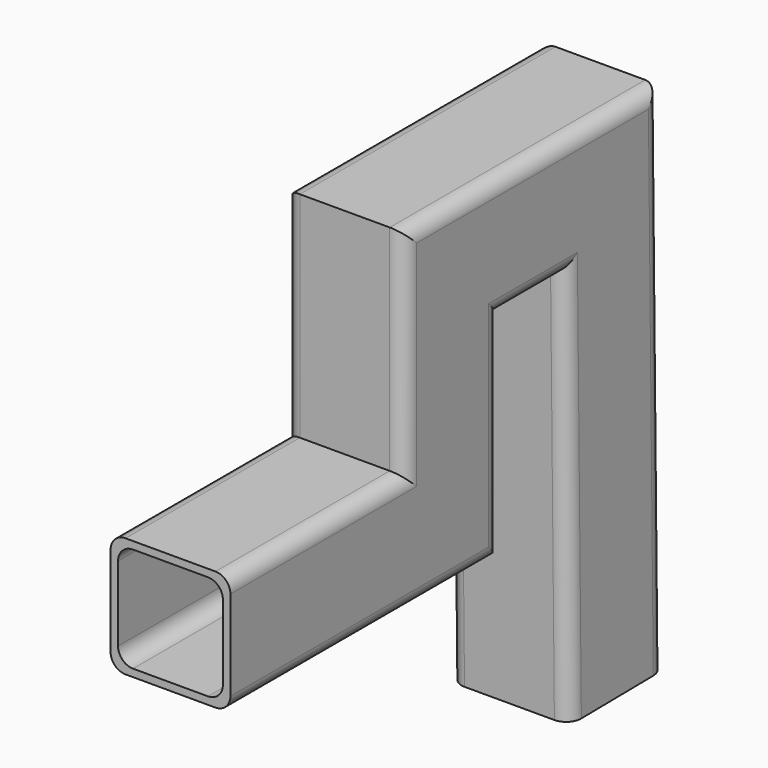
from build123d import *


with BuildPart() as f2:
    # F2: sweep along a path in F1
    with BuildLine(Plane.YZ) as f2_path:
        Line((0, 0), (235.4986518621, 0))
        Line((235.4986518621, 0), (235.4986518621, 181.7011833191))
        Line((235.4986518621, 181.7011833191), (405.3635597229, 181.7011833191))
        Line((405.3635597229, 181.7011833191), (410.0448787212, -205.5106014013))
    # F0 (on Front) → F2 (sweep)
    with BuildSketch(Plane.XZ):
        with BuildLine():
            Line((-43.4998961684, 38.1), (-43.4998961684, -38.1))
            ThreePointArc((-43.4998961684, -38.1), (-39.7801522895, -47.0802561211), (-30.7998961684, -50.8))
            Line((-30.7998961684, -50.8), (45.4001038316, -50.8))
            ThreePointArc((45.4001038316, -50.8), (54.3803599527, -47.0802561211), (58.1001038316, -38.1))
            Line((58.1001038316, -38.1), (58.1001038316, 38.1))
            ThreePointArc((58.1001038316, 38.1), (54.3803599527, 47.0802561211), (45.4001038316, 50.8))
            Line((45.4001038316, 50.8), (-30.7998961684, 50.8))
            ThreePointArc((-30.7998961684, 50.8), (-39.7801522895, 47.0802561211), (-43.4998961684, 38.1))
        make_face()
        with BuildLine():
            ThreePointArc((-37.1498961684, 31.75), (-33.4301522895, 40.7302561211), (-24.4498961684, 44.45))
            Line((-24.4498961684, 44.45), (39.0501038316, 44.45))
            ThreePointArc((39.0501038316, 44.45), (48.0303599527, 40.7302561211), (51.7501038316, 31.75))
            Line((51.7501038316, 31.75), (51.7501038316, -31.75))
            ThreePointArc((51.7501038316, -31.75), (48.0303599527, -40.7302561211), (39.0501038316, -44.45))
            Line((39.0501038316, -44.45), (-24.4498961684, -44.45))
            ThreePointArc((-24.4498961684, -44.45), (-33.4301522895, -40.7302561211), (-37.1498961684, -31.75))
            Line((-37.1498961684, -31.75), (-37.1498961684, 31.75))
        make_face(mode=Mode.SUBTRACT)
    sweep(path=f2_path.line, transition=Transition.RIGHT)


solid = f2.part
